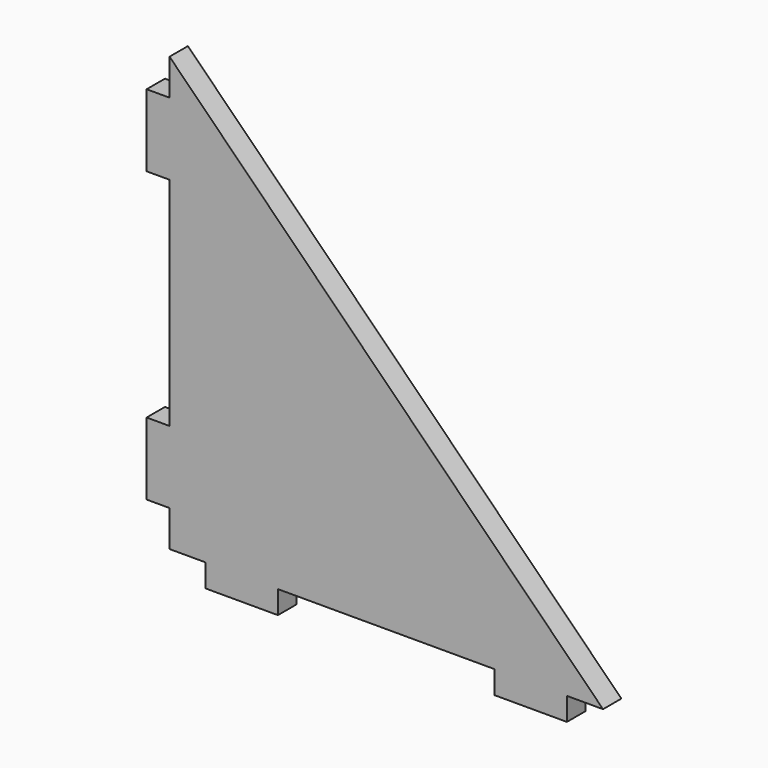
from build123d import *

# Parameters (mm, degrees)
F1_DEPTH = 1.5875


# Not quite as in the source:
# - a length typed as a fraction of an inch, garbled in the dataset ("3 / 203.2 mm" for 3/8 in), is restored


with BuildPart() as f1:
    # F0 (on Front) → F1 (new body)
    with BuildSketch(Plane.XZ):
        Polygon((0, 9.0875), (0, 4.0875), (1.5875, 4.0875), (1.5875, 1.5875), (4.0875, 1.5875), (4.0875, 0), (9.0875, 0), (9.0875, 1.5875), (24.0875, 1.5875), (24.0875, 0), (29.0875, 0), (29.0875, 1.5875), (31.5875, 1.5875), (1.5875, 31.5875), (1.5875, 29.0875), (0, 29.0875), (0, 24.0875), (1.5875, 24.0875), (1.5875, 9.0875), align=None)
    extrude(amount=F1_DEPTH)


solid = f1.part
